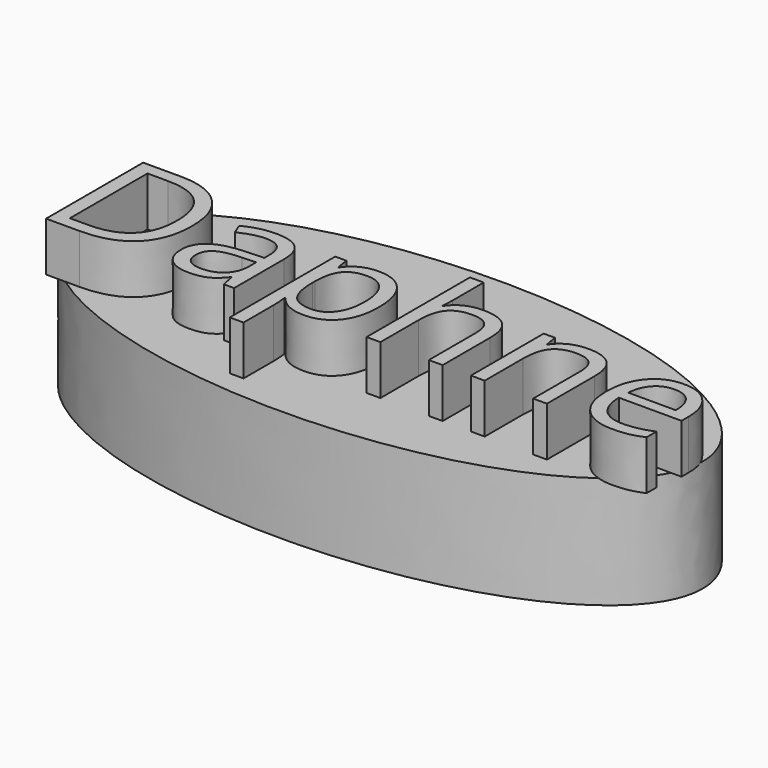
from build123d import *

# Parameters (mm, degrees)
F1_DEPTH     = 25.4
F2_TEXT_SIZE = 38.582399591
F3_DEPTH     = 11.176


# Not quite as in the source:
# - Text() gives the source's letters only with a copy of the font that has no kerning and outlines rounded to 1/6400 em; it was checked with that copy


with BuildPart() as f1:
    # F0 (on Top) → F1 (new body)
    with BuildSketch(Plane.XY):
        with BuildLine():
            add(Edge.make_bspline(
                [(-70.9746554494, 0), (-70.9746554494, -54.8159459085), (35.4873277247, -27.4079729543), (141.9493108988, 0), (35.4873277247, 27.4079729543), (-70.9746554494, 54.8159459085), (-70.9746554494, 0)],
                knots=[0, 0, 0, 2.0943951024, 2.0943951024, 4.1887902048, 4.1887902048, 6.2831853072, 6.2831853072, 6.2831853072], degree=2, weights=[1, 0.5, 1, 0.5, 1, 0.5, 1]))
        make_face()
    extrude(amount=F1_DEPTH)

    # F2 (on face) → F3 (join)
    with BuildSketch(Plane.XY.offset(25.4)):
        with Locations((-68.5325264931, -16.6370710358)):
            Text('Daphne', F2_TEXT_SIZE, font='Open Sans', text_align=(TextAlign.LEFT, TextAlign.BOTTOM))
    extrude(amount=F3_DEPTH)


solid = f1.part
